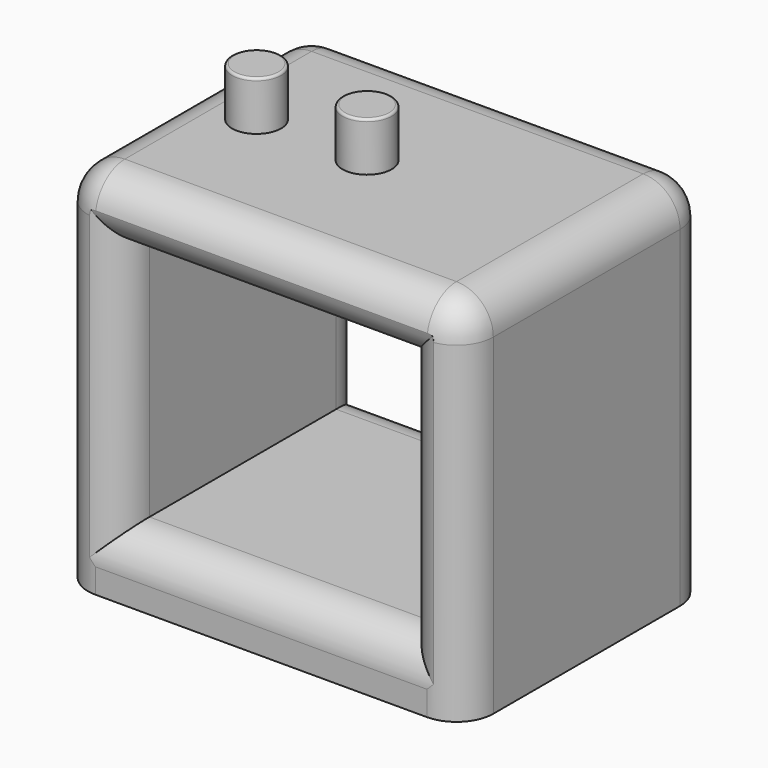
from build123d import *

# Parameters (mm, degrees)
F0_W          = 33
F0_H          = 30
F0_W_2        = 23
F0_H_2        = 20
F1_DEPTH      = 25
F3_DEPTH      = 4
F4_R          = 0.2
F5_T1_DEPTH   = 20
F5_T3_DEPTH   = 23
F5_T5_DEPTH   = 27
F5_T7_DEPTH   = 34.5
F5_T9_DEPTH   = 19
F5_S13_W      = 3
F5_S13_H      = 3
F5_T14_DEPTH  = 3
F5_S19_W      = 3
F5_S19_H      = 3
F5_T20_DEPTH  = 3
F5_S25_W      = 3
F5_S25_H      = 3
F5_T26_DEPTH  = 3
F5_S31_W      = 3
F5_S31_H      = 3
F5_T32_DEPTH  = 3
F5_T39_DEPTH  = 27.5
F5_T43_DEPTH  = 30.5
F5_T50_DEPTH  = 27.5
F5_T54_DEPTH  = 30.5
F5_T61_DEPTH  = 30.5
F5_T65_DEPTH  = 27.5
F5_T72_DEPTH  = 27.5
F5_T76_DEPTH  = 30.5
F5_T83_DEPTH  = 27.5
F5_T87_DEPTH  = 30.5
F5_T94_DEPTH  = 27.5
F5_T98_DEPTH  = 30.5
F5_T105_DEPTH = 30.5
F5_T109_DEPTH = 27.5
F5_T116_DEPTH = 27.5
F5_T120_DEPTH = 30.5


# Not quite as in the source:
# - a fillet or chamfer that OpenCascade refuses, or shapes differently, is made with other operations: its cross-section is extruded or revolved along the edge and cut away or added


with BuildPart() as f1:
    # F0 (on Front) → F1 (new body)
    with BuildSketch(Plane.XZ):
        Rectangle(F0_W, F0_H)
        Rectangle(F0_W_2, F0_H_2, mode=Mode.SUBTRACT)
    extrude(amount=F1_DEPTH)

    # F2 (on face) → F3 (join)
    with BuildSketch(Plane.XY.offset(15)):
        with BuildLine():
            Line((-12.3764710948, -12.5), (-8.3764710948, -12.5))
            ThreePointArc((-8.3764710948, -12.5), (-10.3764710948, -10.5), (-12.3764710948, -12.5))
        make_face()
        with BuildLine():
            ThreePointArc((-12.3764710948, -12.5), (-10.3764710948, -14.5), (-8.3764710948, -12.5))
            Line((-8.3764710948, -12.5), (-12.3764710948, -12.5))
        make_face()
        with BuildLine():
            Line((-3.3764710948, -12.5), (0.6235289052, -12.5))
            ThreePointArc((0.6235289052, -12.5), (-1.3764710948, -10.5), (-3.3764710948, -12.5))
        make_face()
        with BuildLine():
            ThreePointArc((-3.3764710948, -12.5), (-1.3764710948, -14.5), (0.6235289052, -12.5))
            Line((0.6235289052, -12.5), (-3.3764710948, -12.5))
        make_face()
    extrude(amount=F3_DEPTH)

    # F4
    f4_edges = [f1.edges().sort_by_distance(p)[0] for p in [
        (-8.376471, -12.5, 19),
        (0.623529, -12.5, 19),
    ]]
    fillet(f4_edges, radius=F4_R)

    # F5: fillet of radius 3 on 16 edges, made by hand

    # F5_s2 → F5_t1 (cut)
    with BuildSketch(Plane.XY.offset(-10)):
        with BuildLine():
            ThreePointArc((-14.5, -25), (-12.3786796564, -24.1213203436), (-11.5, -22))
            Line((-11.5, -22), (-11.5, -25))
            Line((-11.5, -25), (-14.5, -25))
        make_face()
        with BuildLine():
            ThreePointArc((14.5, -25), (12.3786796564, -24.1213203436), (11.5, -22))
            Line((11.5, -22), (11.5, -25))
            Line((11.5, -25), (14.5, -25))
        make_face()
        with BuildLine():
            ThreePointArc((-14.5, 0), (-12.3786796564, -0.8786796564), (-11.5, -3))
            Line((-11.5, -3), (-11.5, 0))
            Line((-11.5, 0), (-14.5, 0))
        make_face()
        with BuildLine():
            ThreePointArc((14.5, 0), (12.3786796564, -0.8786796564), (11.5, -3))
            Line((11.5, -3), (11.5, 0))
            Line((11.5, 0), (14.5, 0))
        make_face()
    extrude(amount=F5_T1_DEPTH, mode=Mode.SUBTRACT)

    # F5_s4 → F5_t3 (cut)
    with BuildSketch(Plane.YZ.offset(-11.5)):
        with BuildLine():
            ThreePointArc((-25, 13), (-24.1213203436, 10.8786796564), (-22, 10))
            Line((-22, 10), (-25, 10))
            Line((-25, 10), (-25, 13))
        make_face()
        with BuildLine():
            ThreePointArc((-25, -13), (-24.1213203436, -10.8786796564), (-22, -10))
            Line((-22, -10), (-25, -10))
            Line((-25, -10), (-25, -13))
        make_face()
        with BuildLine():
            ThreePointArc((0, 13), (-0.8786796564, 10.8786796564), (-3, 10))
            Line((-3, 10), (0, 10))
            Line((0, 10), (0, 13))
        make_face()
        with BuildLine():
            ThreePointArc((0, -13), (-0.8786796564, -10.8786796564), (-3, -10))
            Line((-3, -10), (0, -10))
            Line((0, -10), (0, -13))
        make_face()
    extrude(amount=F5_T3_DEPTH, mode=Mode.SUBTRACT)

    # F5_s6 → F5_t5 (cut)
    with BuildSketch(Plane.YZ.offset(-13.5)):
        with BuildLine():
            ThreePointArc((-3, 15), (-0.8786796564, 14.1213203436), (0, 12))
            Line((0, 12), (0, 15))
            Line((0, 15), (-3, 15))
        make_face()
        with BuildLine():
            ThreePointArc((-22, 15), (-24.1213203436, 14.1213203436), (-25, 12))
            Line((-25, 12), (-25, 15))
            Line((-25, 15), (-22, 15))
        make_face()
    extrude(amount=F5_T5_DEPTH, mode=Mode.SUBTRACT)

    # F5_s8 → F5_t7 (cut)
    with BuildSketch(Plane.XY.offset(-22.5)):
        with BuildLine():
            ThreePointArc((16.5, -3), (15.6213203436, -0.8786796564), (13.5, 0))
            Line((13.5, 0), (16.5, 0))
            Line((16.5, 0), (16.5, -3))
        make_face()
        with BuildLine():
            ThreePointArc((-13.5, 0), (-15.6213203436, -0.8786796564), (-16.5, -3))
            Line((-16.5, -3), (-16.5, 0))
            Line((-16.5, 0), (-13.5, 0))
        make_face()
        with BuildLine():
            ThreePointArc((-13.5, -25), (-15.6213203436, -24.1213203436), (-16.5, -22))
            Line((-16.5, -22), (-16.5, -25))
            Line((-16.5, -25), (-13.5, -25))
        make_face()
        with BuildLine():
            ThreePointArc((16.5, -22), (15.6213203436, -24.1213203436), (13.5, -25))
            Line((13.5, -25), (16.5, -25))
            Line((16.5, -25), (16.5, -22))
        make_face()
    extrude(amount=F5_T7_DEPTH, mode=Mode.SUBTRACT)

    # F5_s10 → F5_t9 (cut)
    with BuildSketch(Plane.XZ.offset(3)):
        with BuildLine():
            ThreePointArc((-13.5, 15), (-15.6213203436, 14.1213203436), (-16.5, 12))
            Line((-16.5, 12), (-16.5, 15))
            Line((-16.5, 15), (-13.5, 15))
        make_face()
        with BuildLine():
            ThreePointArc((13.5, 15), (15.6213203436, 14.1213203436), (16.5, 12))
            Line((16.5, 12), (16.5, 15))
            Line((16.5, 15), (13.5, 15))
        make_face()
    extrude(amount=F5_T9_DEPTH, mode=Mode.SUBTRACT)


with BuildPart() as f5_tool12:
    # F5_s13 → F5_t14 (new body)
    with BuildSketch(Plane.XY.offset(12)):
        with Locations((15, -1.5)):
            Rectangle(F5_S13_W, F5_S13_H)
    extrude(amount=F5_T14_DEPTH)

    # F5_s15 → F5_t16 (revolve, cut)
    with BuildSketch(Plane(origin=(13.5, -3, 12), x_dir=(-0.7071067812, -0.7071067812, 0), z_dir=(-0.7071067812, 0.7071067812, 0))):
        with BuildLine():
            ThreePointArc((0, -3), (3, 0), (0, 3))
            Line((0, 3), (0, -3))
        make_face()
    revolve(axis=Axis((13.5, -3, 12), (0, 0, 1)), mode=Mode.SUBTRACT)


with BuildPart() as f1_1:
    add(f1.part)

    # F5_t11: cut F5_tool12
    add(f5_tool12.part, mode=Mode.SUBTRACT)


with BuildPart() as f5_tool18:
    # F5_s19 → F5_t20 (new body)
    with BuildSketch(Plane.XY.offset(12)):
        with Locations((-15, -1.5)):
            Rectangle(F5_S19_W, F5_S19_H)
    extrude(amount=F5_T20_DEPTH)

    # F5_s21 → F5_t22 (revolve, cut)
    with BuildSketch(Plane(origin=(-13.5, -3, 12), x_dir=(0.7071067812, -0.7071067812, 0), z_dir=(-0.7071067812, -0.7071067812, 0))):
        with BuildLine():
            ThreePointArc((0, -3), (3, 0), (0, 3))
            Line((0, 3), (0, -3))
        make_face()
    revolve(axis=Axis((-13.5, -3, 12), (0, 0, 1)), mode=Mode.SUBTRACT)


with BuildPart() as f1_2:
    add(f1_1.part)

    # F5_t17: cut F5_tool18
    add(f5_tool18.part, mode=Mode.SUBTRACT)


with BuildPart() as f5_tool24:
    # F5_s25 → F5_t26 (new body)
    with BuildSketch(Plane.XY.offset(12)):
        with Locations((-15, -23.5)):
            Rectangle(F5_S25_W, F5_S25_H)
    extrude(amount=F5_T26_DEPTH)

    # F5_s27 → F5_t28 (revolve, cut)
    with BuildSketch(Plane(origin=(-13.5, -22, 12), x_dir=(0.7071067812, 0.7071067812, 0), z_dir=(0.7071067812, -0.7071067812, 0))):
        with BuildLine():
            ThreePointArc((0, -3), (3, 0), (0, 3))
            Line((0, 3), (0, -3))
        make_face()
    revolve(axis=Axis((-13.5, -22, 12), (0, 0, 1)), mode=Mode.SUBTRACT)


with BuildPart() as f1_3:
    add(f1_2.part)

    # F5_t23: cut F5_tool24
    add(f5_tool24.part, mode=Mode.SUBTRACT)


with BuildPart() as f5_tool30:
    # F5_s31 → F5_t32 (new body)
    with BuildSketch(Plane.XY.offset(12)):
        with Locations((15, -23.5)):
            Rectangle(F5_S31_W, F5_S31_H)
    extrude(amount=F5_T32_DEPTH)

    # F5_s33 → F5_t34 (revolve, cut)
    with BuildSketch(Plane(origin=(13.5, -22, 12), x_dir=(-0.7071067812, 0.7071067812, 0), z_dir=(0.7071067812, 0.7071067812, 0))):
        with BuildLine():
            ThreePointArc((0, -3), (3, 0), (0, 3))
            Line((0, 3), (0, -3))
        make_face()
    revolve(axis=Axis((13.5, -22, 12), (0, 0, 1)), mode=Mode.SUBTRACT)


with BuildPart() as f1_4:
    add(f1_3.part)

    # F5_t29: cut F5_tool30
    add(f5_tool30.part, mode=Mode.SUBTRACT)


with BuildPart() as f5_tool37:
    # F5_s38 → F5_t39 (new body)
    with BuildSketch(Plane.XY.offset(-17.5)):
        with BuildLine():
            ThreePointArc((-14.5, -25), (-12.3786796564, -24.1213203436), (-11.5, -22))
            Line((-11.5, -22), (-11.5, -25))
            Line((-11.5, -25), (-14.5, -25))
        make_face()
    extrude(amount=F5_T39_DEPTH)

    split(bisect_by=Plane.XY.offset(-10), keep=Keep.BOTTOM)


with BuildPart() as f5_tool41:
    # F5_s42 → F5_t43 (new body)
    with BuildSketch(Plane.YZ.offset(11.5)):
        with BuildLine():
            ThreePointArc((-25, -13), (-24.1213203436, -10.8786796564), (-22, -10))
            Line((-22, -10), (-25, -10))
            Line((-25, -10), (-25, -13))
        make_face()
    extrude(amount=-F5_T43_DEPTH)

    split(bisect_by=Plane.YZ.offset(-11.5), keep=Keep.BOTTOM)


with BuildPart() as f5_tool37_1:
    add(f5_tool37.part)

    # F5_t45: intersect F5_tool41
    add(f5_tool41.part, mode=Mode.INTERSECT)


with BuildPart() as f1_5:
    add(f1_4.part)

    # F5_t35: cut F5_tool37
    add(f5_tool37_1.part, mode=Mode.SUBTRACT)


with BuildPart() as f5_tool48:
    # F5_s49 → F5_t50 (new body)
    with BuildSketch(Plane.XY.offset(-10)):
        with BuildLine():
            ThreePointArc((-14.5, -25), (-12.3786796564, -24.1213203436), (-11.5, -22))
            Line((-11.5, -22), (-11.5, -25))
            Line((-11.5, -25), (-14.5, -25))
        make_face()
    extrude(amount=F5_T50_DEPTH)

    split(bisect_by=Plane.XY.offset(10), keep=Keep.TOP)


with BuildPart() as f5_tool52:
    # F5_s53 → F5_t54 (new body)
    with BuildSketch(Plane.YZ.offset(-19)):
        with BuildLine():
            ThreePointArc((-25, 13), (-24.1213203436, 10.8786796564), (-22, 10))
            Line((-22, 10), (-25, 10))
            Line((-25, 10), (-25, 13))
        make_face()
    extrude(amount=F5_T54_DEPTH)

    split(bisect_by=Plane.YZ.offset(-11.5), keep=Keep.BOTTOM)


with BuildPart() as f5_tool48_1:
    add(f5_tool48.part)

    # F5_t56: intersect F5_tool52
    add(f5_tool52.part, mode=Mode.INTERSECT)


with BuildPart() as f1_6:
    add(f1_5.part)

    # F5_t46: cut F5_tool48
    add(f5_tool48_1.part, mode=Mode.SUBTRACT)


with BuildPart() as f5_tool59:
    # F5_s60 → F5_t61 (new body)
    with BuildSketch(Plane.YZ.offset(-11.5)):
        with BuildLine():
            ThreePointArc((-25, 13), (-24.1213203436, 10.8786796564), (-22, 10))
            Line((-22, 10), (-25, 10))
            Line((-25, 10), (-25, 13))
        make_face()
    extrude(amount=F5_T61_DEPTH)

    split(bisect_by=Plane.YZ.offset(11.5), keep=Keep.TOP)


with BuildPart() as f5_tool63:
    # F5_s64 → F5_t65 (new body)
    with BuildSketch(Plane.XY.offset(17.5)):
        with BuildLine():
            ThreePointArc((14.5, -25), (12.3786796564, -24.1213203436), (11.5, -22))
            Line((11.5, -22), (11.5, -25))
            Line((11.5, -25), (14.5, -25))
        make_face()
    extrude(amount=-F5_T65_DEPTH)

    split(bisect_by=Plane.XY.offset(10), keep=Keep.TOP)


with BuildPart() as f5_tool59_1:
    add(f5_tool59.part)

    # F5_t67: intersect F5_tool63
    add(f5_tool63.part, mode=Mode.INTERSECT)


with BuildPart() as f1_7:
    add(f1_6.part)

    # F5_t57: cut F5_tool59
    add(f5_tool59_1.part, mode=Mode.SUBTRACT)


with BuildPart() as f5_tool70:
    # F5_s71 → F5_t72 (new body)
    with BuildSketch(Plane.XY.offset(10)):
        with BuildLine():
            ThreePointArc((14.5, -25), (12.3786796564, -24.1213203436), (11.5, -22))
            Line((11.5, -22), (11.5, -25))
            Line((11.5, -25), (14.5, -25))
        make_face()
    extrude(amount=-F5_T72_DEPTH)

    split(bisect_by=Plane.XY.offset(-10), keep=Keep.BOTTOM)


with BuildPart() as f5_tool74:
    # F5_s75 → F5_t76 (new body)
    with BuildSketch(Plane.YZ.offset(19)):
        with BuildLine():
            ThreePointArc((-25, -13), (-24.1213203436, -10.8786796564), (-22, -10))
            Line((-22, -10), (-25, -10))
            Line((-25, -10), (-25, -13))
        make_face()
    extrude(amount=-F5_T76_DEPTH)

    split(bisect_by=Plane.YZ.offset(11.5), keep=Keep.TOP)


with BuildPart() as f5_tool70_1:
    add(f5_tool70.part)

    # F5_t78: intersect F5_tool74
    add(f5_tool74.part, mode=Mode.INTERSECT)


with BuildPart() as f1_8:
    add(f1_7.part)

    # F5_t68: cut F5_tool70
    add(f5_tool70_1.part, mode=Mode.SUBTRACT)


with BuildPart() as f5_tool81:
    # F5_s82 → F5_t83 (new body)
    with BuildSketch(Plane.XY.offset(-17.5)):
        with BuildLine():
            ThreePointArc((-14.5, 0), (-12.3786796564, -0.8786796564), (-11.5, -3))
            Line((-11.5, -3), (-11.5, 0))
            Line((-11.5, 0), (-14.5, 0))
        make_face()
    extrude(amount=F5_T83_DEPTH)

    split(bisect_by=Plane.XY.offset(-10), keep=Keep.BOTTOM)


with BuildPart() as f5_tool85:
    # F5_s86 → F5_t87 (new body)
    with BuildSketch(Plane.YZ.offset(11.5)):
        with BuildLine():
            ThreePointArc((0, -13), (-0.8786796564, -10.8786796564), (-3, -10))
            Line((-3, -10), (0, -10))
            Line((0, -10), (0, -13))
        make_face()
    extrude(amount=-F5_T87_DEPTH)

    split(bisect_by=Plane.YZ.offset(-11.5), keep=Keep.BOTTOM)


with BuildPart() as f5_tool81_1:
    add(f5_tool81.part)

    # F5_t89: intersect F5_tool85
    add(f5_tool85.part, mode=Mode.INTERSECT)


with BuildPart() as f1_9:
    add(f1_8.part)

    # F5_t79: cut F5_tool81
    add(f5_tool81_1.part, mode=Mode.SUBTRACT)


with BuildPart() as f5_tool92:
    # F5_s93 → F5_t94 (new body)
    with BuildSketch(Plane.XY.offset(-10)):
        with BuildLine():
            ThreePointArc((-14.5, 0), (-12.3786796564, -0.8786796564), (-11.5, -3))
            Line((-11.5, -3), (-11.5, 0))
            Line((-11.5, 0), (-14.5, 0))
        make_face()
    extrude(amount=F5_T94_DEPTH)

    split(bisect_by=Plane.XY.offset(10), keep=Keep.TOP)


with BuildPart() as f5_tool96:
    # F5_s97 → F5_t98 (new body)
    with BuildSketch(Plane.YZ.offset(-19)):
        with BuildLine():
            ThreePointArc((0, 13), (-0.8786796564, 10.8786796564), (-3, 10))
            Line((-3, 10), (0, 10))
            Line((0, 10), (0, 13))
        make_face()
    extrude(amount=F5_T98_DEPTH)

    split(bisect_by=Plane.YZ.offset(-11.5), keep=Keep.BOTTOM)


with BuildPart() as f5_tool92_1:
    add(f5_tool92.part)

    # F5_t100: intersect F5_tool96
    add(f5_tool96.part, mode=Mode.INTERSECT)


with BuildPart() as f1_10:
    add(f1_9.part)

    # F5_t90: cut F5_tool92
    add(f5_tool92_1.part, mode=Mode.SUBTRACT)


with BuildPart() as f5_tool103:
    # F5_s104 → F5_t105 (new body)
    with BuildSketch(Plane.YZ.offset(-11.5)):
        with BuildLine():
            ThreePointArc((0, 13), (-0.8786796564, 10.8786796564), (-3, 10))
            Line((-3, 10), (0, 10))
            Line((0, 10), (0, 13))
        make_face()
    extrude(amount=F5_T105_DEPTH)

    split(bisect_by=Plane.YZ.offset(11.5), keep=Keep.TOP)


with BuildPart() as f5_tool107:
    # F5_s108 → F5_t109 (new body)
    with BuildSketch(Plane.XY.offset(17.5)):
        with BuildLine():
            ThreePointArc((14.5, 0), (12.3786796564, -0.8786796564), (11.5, -3))
            Line((11.5, -3), (11.5, 0))
            Line((11.5, 0), (14.5, 0))
        make_face()
    extrude(amount=-F5_T109_DEPTH)

    split(bisect_by=Plane.XY.offset(10), keep=Keep.TOP)


with BuildPart() as f5_tool103_1:
    add(f5_tool103.part)

    # F5_t111: intersect F5_tool107
    add(f5_tool107.part, mode=Mode.INTERSECT)


with BuildPart() as f1_11:
    add(f1_10.part)

    # F5_t101: cut F5_tool103
    add(f5_tool103_1.part, mode=Mode.SUBTRACT)


with BuildPart() as f5_tool114:
    # F5_s115 → F5_t116 (new body)
    with BuildSketch(Plane.XY.offset(10)):
        with BuildLine():
            ThreePointArc((14.5, 0), (12.3786796564, -0.8786796564), (11.5, -3))
            Line((11.5, -3), (11.5, 0))
            Line((11.5, 0), (14.5, 0))
        make_face()
    extrude(amount=-F5_T116_DEPTH)

    split(bisect_by=Plane.XY.offset(-10), keep=Keep.BOTTOM)


with BuildPart() as f5_tool118:
    # F5_s119 → F5_t120 (new body)
    with BuildSketch(Plane.YZ.offset(19)):
        with BuildLine():
            ThreePointArc((0, -13), (-0.8786796564, -10.8786796564), (-3, -10))
            Line((-3, -10), (0, -10))
            Line((0, -10), (0, -13))
        make_face()
    extrude(amount=-F5_T120_DEPTH)

    split(bisect_by=Plane.YZ.offset(11.5), keep=Keep.TOP)


with BuildPart() as f5_tool114_1:
    add(f5_tool114.part)

    # F5_t122: intersect F5_tool118
    add(f5_tool118.part, mode=Mode.INTERSECT)


with BuildPart() as f1_12:
    add(f1_11.part)

    # F5_t112: cut F5_tool114
    add(f5_tool114_1.part, mode=Mode.SUBTRACT)


solid = f1_12.part
